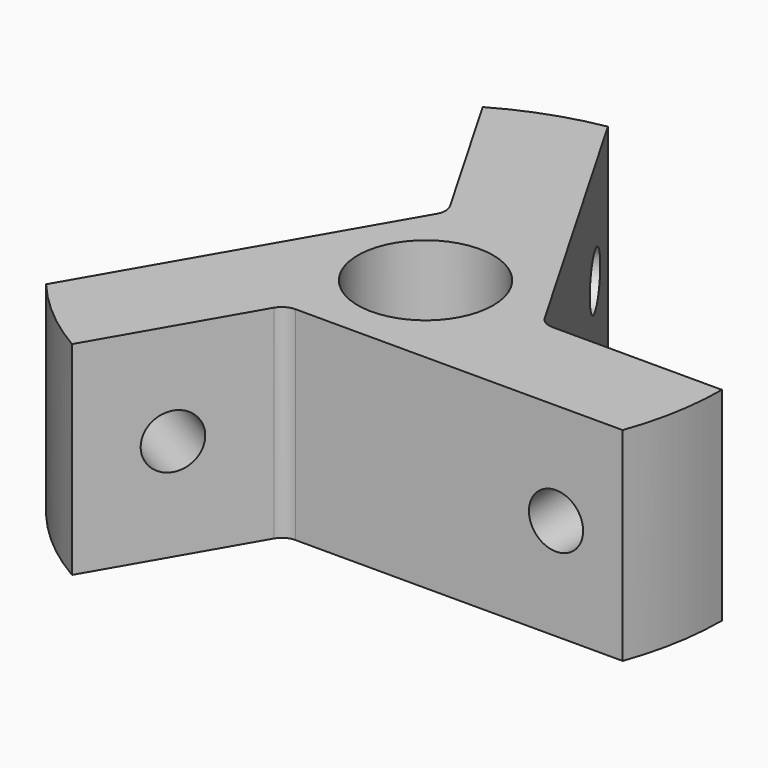
from build123d import *

# Parameters (mm, degrees)
F0_R            = 4
F1_DEPTH        = 12
F3_D            = 3.2
F3_DEPTH        = 6
F3_TIP          = 0.9613769904
F3_COPIES_COUNT = 3


# Not quite as in the source:
# - a pattern or mirror of a feature is missing from the dataset's text; its kind, count and spacing are read off the source's solid


with BuildPart() as f1:
    # F0 (on Top) → F1 (new body)
    with BuildSketch(Plane.XY):
        with BuildLine():
            Line((-2.8867513459, -6), (16.4392822228, -6))
            ThreePointArc((16.4392822228, -6), (17.2327803749, -3.0465194158), (17.5, 0))
            Line((17.5, 0), (7.5055534995, 0))
            ThreePointArc((7.5055534995, 0), (7.0055534995, 0.1339745962), (6.6395280957, 0.5))
            Line((6.6395280957, 0.5), (-3.0234886887, 17.2368360249))
            ThreePointArc((-3.0234886887, 17.2368360249), (-5.9780269803, 16.4472852904), (-8.75, 15.1554445662))
            Line((-8.75, 15.1554445662), (-3.7527767497, 6.5))
            ThreePointArc((-3.7527767497, 6.5), (-3.6188021535, 6), (-3.7527767497, 5.5))
            Line((-3.7527767497, 5.5), (-13.4157935341, -11.2368360249))
            ThreePointArc((-13.4157935341, -11.2368360249), (-11.2547533946, -13.4007658746), (-8.75, -15.1554445662))
            Line((-8.75, -15.1554445662), (-3.7527767497, -6.5))
            ThreePointArc((-3.7527767497, -6.5), (-3.3867513459, -6.1339745962), (-2.8867513459, -6))
        make_face()
        Circle(F0_R, mode=Mode.SUBTRACT)
    extrude(amount=F1_DEPTH)

    # F3
    with Locations(Plane(origin=(0, 0, 0), x_dir=(-1, 0, 0), z_dir=(0, 1, 0))):
        with Locations((-12.5027767497, 6)):
            f3 = Hole(F3_D / 2, depth=F3_DEPTH)
            with Locations((0, 0, -(F3_DEPTH + F3_TIP / 2))):  # 118° drill point
                Cone(0, F3_D / 2, F3_TIP, mode=Mode.SUBTRACT)

    # F3_copies: F3 ×3 about axis
    f3_copies_axis = Axis((0, 0, 0), (0, 0, 1))
    for i in range(1, F3_COPIES_COUNT):
        add(f3.rotate(f3_copies_axis, i * 360 / F3_COPIES_COUNT), mode=Mode.SUBTRACT)


solid = f1.part
